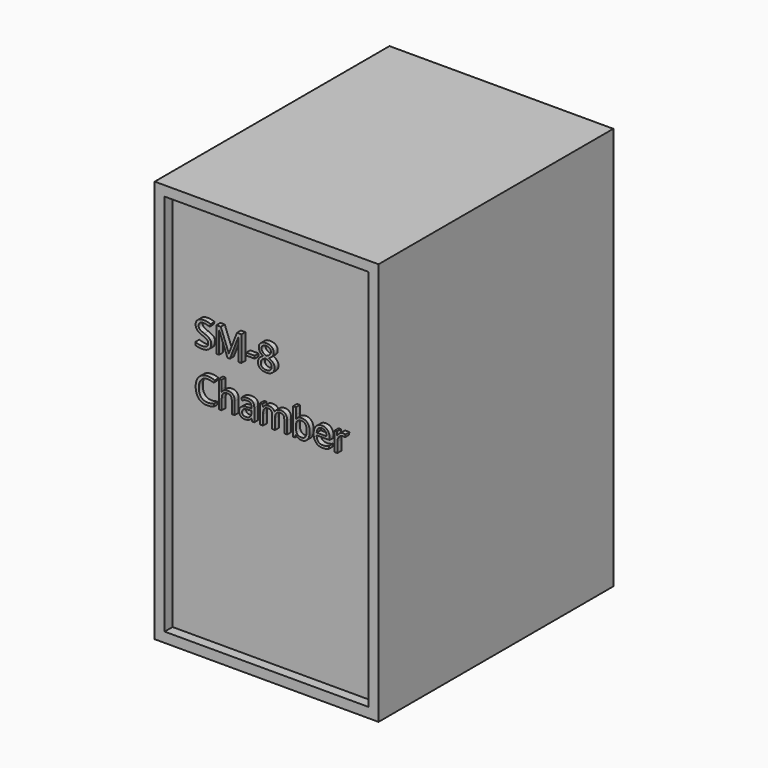
from build123d import *

# Parameters (mm, degrees)
F0_W         = 1143
F0_H         = 1498.6
F1_DEPTH     = 2057.4
F2_W         = 1041.4
F2_H         = 1955.8
F3_DEPTH     = 50.8
F4_TEXT_SIZE = 180.4411343455
F5_DEPTH     = 25.4


# Not quite as in the source:
# - Text() gives the source's letters only with a copy of the font that has no kerning and outlines rounded to 1/6400 em; it was checked with that copy


with BuildPart() as f1:
    # F0 (on Top) → F1 (new body)
    with BuildSketch(Plane.XY):
        Rectangle(F0_W, F0_H)
    extrude(amount=F1_DEPTH)

    # F2 (on face) → F3 (cut)
    with BuildSketch(Plane.XZ.offset(749.3)):
        with Locations((0, 1028.7)):
            Rectangle(F2_W, F2_H)
    extrude(amount=-F3_DEPTH, mode=Mode.SUBTRACT)

    # F4 (on face) → F5 (join)
    with BuildSketch(Plane.XZ.offset(698.5)):
        with Locations((-393.7, 1368.6823832713)):
            Text('SM-8', F4_TEXT_SIZE, font='Open Sans', text_align=(TextAlign.LEFT, TextAlign.BOTTOM))
        with Locations((-393.7, 1123.2824405614)):
            Text('Chamber', F4_TEXT_SIZE, font='Open Sans', text_align=(TextAlign.LEFT, TextAlign.BOTTOM))
    extrude(amount=F5_DEPTH)


solid = f1.part
